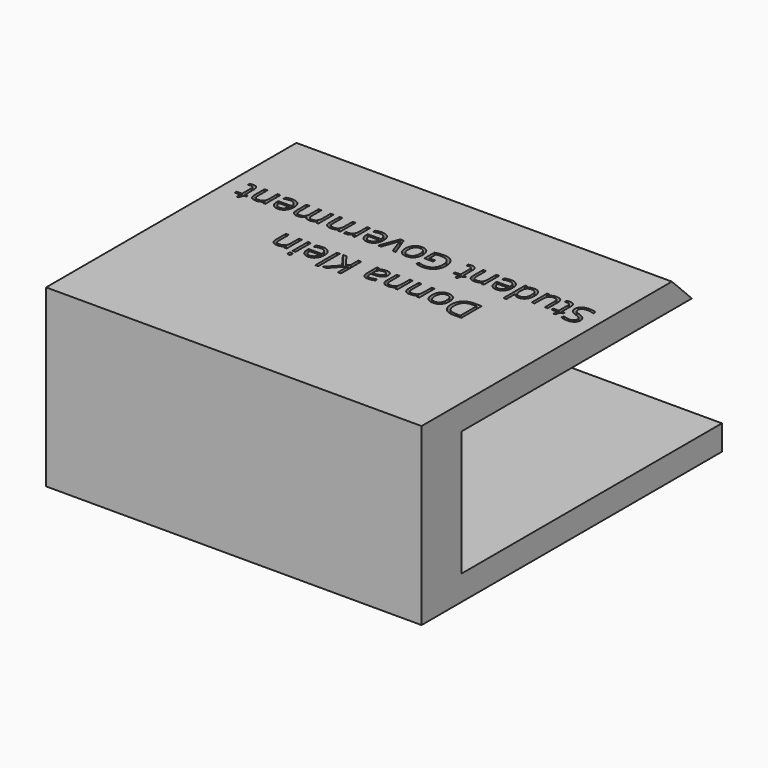
from build123d import *

# Parameters (mm, degrees)
F0_W           = 76.2
F0_H           = 76.2
F1_DEPTH       = 5.08
F2_W           = 76.2
F2_H           = 10.16
F3_DEPTH       = 25.4
F4_W           = 76.2
F4_H           = 66.04
F4_H_2         = 10.16
F5_DEPTH       = 5.08
F6_T1_DEPTH    = 141.5207478943
F7_TEXT_SIZE   = 7.2320061012
F8_DEPTH       = 2.54
F9_TEXT_SIZE   = 66.7506159321
F9_TEXT_SIZE_2 = 7.1557169583
F10_DEPTH      = 1.905


# Not quite as in the source:
# - a fillet or chamfer that OpenCascade refuses, or shapes differently, is made with other operations: its cross-section is extruded or revolved along the edge and cut away or added
# - Text() gives the source's letters only with a copy of the font that has no kerning and outlines rounded to 1/6400 em; it was checked with that copy


with BuildPart() as f1:
    # F0 (on Top) → F1 (new body)
    with BuildSketch(Plane.XY):
        Rectangle(F0_W, F0_H)
    extrude(amount=F1_DEPTH)

    # F2 (on face) → F3 (join)
    with BuildSketch(Plane.XY.offset(5.08)):
        with Locations((0, -33.02)):
            Rectangle(F2_W, F2_H)
    extrude(amount=F3_DEPTH)

    # F4 (on face) → F5 (join)
    with BuildSketch(Plane.XY.offset(30.48)):
        with Locations((0, 5.08)):
            Rectangle(F4_W, F4_H)
        with Locations((0, -33.02)):
            Rectangle(F4_W, F4_H_2)
    extrude(amount=F5_DEPTH)

    # F6: chamfer of 12.7 on 1 edges, made by hand

    # F6_s2 → F6_t1 (cut)
    with BuildSketch(Plane.YZ.offset(-70.7603739472)):
        Polygon((38.1, 22.86), (25.4, 35.56), (38.1, 35.56), align=None)
    extrude(amount=F6_T1_DEPTH, mode=Mode.SUBTRACT)

    # F7 (on face) → F8 (cut)
    with BuildSketch(Plane.XY.offset(35.56)):
        with Locations(Location((20.526467317, 0), (0, 0, -180))):
            Text('Donna Klein', F7_TEXT_SIZE, font='Open Sans', text_align=(TextAlign.LEFT, TextAlign.BOTTOM))
        with Locations(Location((35.56, 9.8355282977), (0, 0, -180))):
            Text('Student Government', F7_TEXT_SIZE, font='Open Sans', text_align=(TextAlign.LEFT, TextAlign.BOTTOM))
    extrude(amount=-F8_DEPTH, mode=Mode.SUBTRACT)

    # F9 (on face) → F10 (cut)
    with BuildSketch(Plane(origin=(0, 0, 0), x_dir=(1, 0, 0), z_dir=(0, 0, -1))):
        with Locations((-19.05, -24.0302161)):
            Text('$', F9_TEXT_SIZE, font='Open Sans', text_align=(TextAlign.LEFT, TextAlign.BOTTOM))
        with Locations((-35.56, -35.56)):
            Text('NR', F9_TEXT_SIZE_2, font='Open Sans', text_align=(TextAlign.LEFT, TextAlign.BOTTOM))
    extrude(amount=-F10_DEPTH, mode=Mode.SUBTRACT)


solid = f1.part
